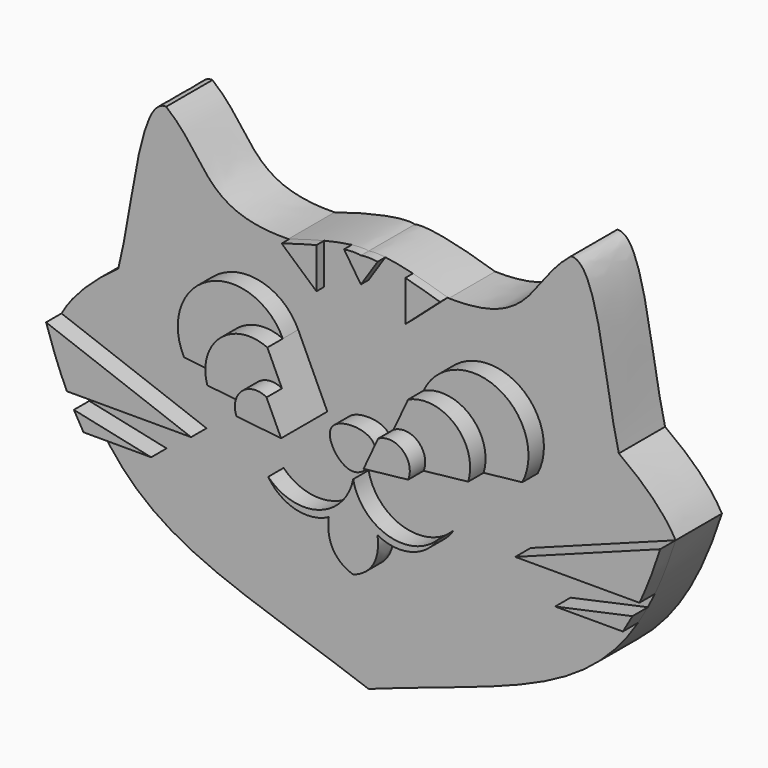
from build123d import *

# Parameters (mm, degrees)
F1_DEPTH       = 7.62
F3_DEPTH       = 2.54
F5_DEPTH       = 2.54
F7_DEPTH       = 2.54
F9_DEPTH       = 2.54
F10_DEPTH      = 1.27
F11_R          = 6.1705322235
F12_DEPTH      = 25.4
F12_DEPTH_BACK = 40.9956
F15_DEPTH      = 2.54
F16_DEPTH      = 2.54
F17_DEPTH      = 2.54


# Not quite as in the source:
# - a feature of the source that left no trace in its solid (it failed there, or was rolled back) is left out


with BuildPart() as f1:
    # F0 (on Front) → F1 (new body)
    with BuildSketch(Plane.XZ):
        with BuildLine():
            add(Edge.make_bspline(
                [(0, 20.3936955137), (1.3948995364, 20.766500107), (5.4805992876, 19.9818174569), (10.5812398311, 18.3488156712)],
                knots=[0, 0, 0, 0, 14.7407470762, 14.7407470762, 14.7407470762, 14.7407470762], degree=3))
            add(Edge.make_bspline(
                [(0, 20.3936955137), (-1.3948995364, 20.766500107), (-5.4805992876, 19.9818174569), (-10.5812398311, 18.3488156712)],
                knots=[0, 0, 0, 0, 14.7407470762, 14.7407470762, 14.7407470762, 14.7407470762], degree=3))
            add(Edge.make_bspline(
                [(-10.5812398311, 18.3488156712), (-17.5782727848, 16.1086720636), (-26.4852430335, 12.2721433588), (-32.9759645779, 7.637338707)],
                knots=[14.7407470762, 14.7407470762, 14.7407470762, 14.7407470762, 34.9620295163, 34.9620295163, 34.9620295163, 34.9620295163], degree=3))
            add(Edge.make_bspline(
                [(-32.9759645779, 7.637338707), (-36.2982275011, 5.2650231569), (-38.9874613211, 2.6835685783), (-40.4635321278, 0)],
                knots=[34.9620295163, 34.9620295163, 34.9620295163, 34.9620295163, 45.3122527465, 45.3122527465, 45.3122527465, 45.3122527465], degree=3))
            add(Edge.make_bspline(
                [(-40.4635321278, 0), (-33.4182982388, -22.0806543438), (-22.6069154368, -22.2432924496), (0, -30.4063044863)],
                knots=[0, 0, 0, 0, 50.6146301455, 50.6146301455, 50.6146301455, 50.6146301455], degree=3))
            add(Edge.make_bspline(
                [(40.4635321278, 0), (33.4182982388, -22.0806543438), (22.6069154368, -22.2432924496), (0, -30.4063044863)],
                knots=[0, 0, 0, 0, 50.6146301455, 50.6146301455, 50.6146301455, 50.6146301455], degree=3))
            add(Edge.make_bspline(
                [(32.9759645779, 7.637338707), (36.2982275011, 5.2650231569), (38.9874613211, 2.6835685783), (40.4635321278, 0)],
                knots=[34.9620295163, 34.9620295163, 34.9620295163, 34.9620295163, 45.3122527465, 45.3122527465, 45.3122527465, 45.3122527465], degree=3))
            add(Edge.make_bspline(
                [(10.5812398311, 18.3488156712), (17.5782727848, 16.1086720636), (26.4852430335, 12.2721433588), (32.9759645779, 7.637338707)],
                knots=[14.7407470762, 14.7407470762, 14.7407470762, 14.7407470762, 34.9620295163, 34.9620295163, 34.9620295163, 34.9620295163], degree=3))
        make_face()
        with BuildLine():
            add(Edge.make_bspline(
                [(-10.5812398311, 18.3488156712), (-17.5782727848, 16.1086720636), (-26.4852430335, 12.2721433588), (-32.9759645779, 7.637338707)],
                knots=[14.7407470762, 14.7407470762, 14.7407470762, 14.7407470762, 34.9620295163, 34.9620295163, 34.9620295163, 34.9620295163], degree=3))
            add(Edge.make_bspline(
                [(-26.6729070635, 28.4619446353), (-21.143157325, 24.0706735486), (-21.7953124032, 18.1571517645), (-10.5812398311, 18.3488156712)],
                knots=[0, 0, 0, 0, 19.0057131348, 19.0057131348, 19.0057131348, 19.0057131348], degree=3))
            add(Edge.make_bspline(
                [(-32.9759645779, 7.637338707), (-31.0729775939, 15.0011911106), (-30.2509800414, 28.7872230125), (-26.6729070635, 28.4619446353)],
                knots=[0, 0, 0, 0, 21.7575905399, 21.7575905399, 21.7575905399, 21.7575905399], degree=3))
        make_face()
        with BuildLine():
            add(Edge.make_bspline(
                [(26.6729070635, 28.4619446353), (21.143157325, 24.0706735486), (21.7953124032, 18.1571517645), (10.5812398311, 18.3488156712)],
                knots=[0, 0, 0, 0, 19.0057131348, 19.0057131348, 19.0057131348, 19.0057131348], degree=3))
            add(Edge.make_bspline(
                [(10.5812398311, 18.3488156712), (17.5782727848, 16.1086720636), (26.4852430335, 12.2721433588), (32.9759645779, 7.637338707)],
                knots=[14.7407470762, 14.7407470762, 14.7407470762, 14.7407470762, 34.9620295163, 34.9620295163, 34.9620295163, 34.9620295163], degree=3))
            add(Edge.make_bspline(
                [(32.9759645779, 7.637338707), (31.0729775939, 15.0011911106), (30.2509800414, 28.7872230125), (26.6729070635, 28.4619446353)],
                knots=[0, 0, 0, 0, 21.7575905399, 21.7575905399, 21.7575905399, 21.7575905399], degree=3))
        make_face()
    extrude(amount=F1_DEPTH)

    # F2 (on face) → F3 (join)
    with BuildSketch(Plane.XZ.offset(7.62)):
        with BuildLine():
            Line((-22.2900346122, 1.8519903891), (-5.4355557593, 0))
            Line((-5.4355557593, 0), (-9.2711227015, 8.2497525646))
            ThreePointArc((-9.2711227015, 8.2497525646), (-19.0491804333, 11.7022032129), (-22.2900346122, 1.8519903891))
        make_face()
        with BuildLine():
            Line((9.2711227015, 8.2497525646), (5.4355557593, 0))
            Line((5.4355557593, 0), (22.2900346122, 1.8519903891))
            ThreePointArc((22.2900346122, 1.8519903891), (19.0491804333, 11.7022032129), (9.2711227015, 8.2497525646))
        make_face()
        with BuildLine():
            add(Edge.make_bspline(
                [(-2.8783681854, 0), (-2.0189454867, 1.4877631411), (5.432970272, 1.496369958), (0.0323743257, -6.8934681979), (-3.6948527353, -1.4134320869), (-2.8783681854, 0)],
                knots=[0, 0, 0, 0, 0.3458251097, 0.6714528725, 1, 1, 1, 1], degree=3))
        make_face()
    extrude(amount=F3_DEPTH)

    # F4 (on face) → F5 (join)
    with BuildSketch(Plane.XZ.offset(10.16)):
        with BuildLine():
            Line((-5.4355557593, 0), (-9.2711227015, 8.2497525646))
            ThreePointArc((-9.2711227015, 8.2497525646), (-15.4885144267, 7.3406406044), (-17.1882661896, 1.2914019444))
            Line((-17.1882661896, 1.2914019444), (-5.4355557593, 0))
        make_face()
        with BuildLine():
            ThreePointArc((17.1882661896, 1.2914019444), (15.4885144267, 7.3406406044), (9.2711227015, 8.2497525646))
            Line((9.2711227015, 8.2497525646), (5.4355557593, 0))
            Line((5.4355557593, 0), (17.1882661896, 1.2914019444))
        make_face()
    extrude(amount=F5_DEPTH)

    # F6 (on face) → F7 (join)
    with BuildSketch(Plane.XZ.offset(12.7)):
        with BuildLine():
            Line((-5.4355557593, 0), (-7.3533392304, 4.1248762823))
            ThreePointArc((-7.3533392304, 4.1248762823), (-10.5856202932, 3.810934338), (-11.3119109744, 0.6457009722))
            Line((-11.3119109744, 0.6457009722), (-5.4355557593, 0))
        make_face()
        with BuildLine():
            ThreePointArc((11.3119109744, 0.6457009722), (10.5856202932, 3.810934338), (7.3533392304, 4.1248762823))
            Line((7.3533392304, 4.1248762823), (5.4355557593, 0))
            Line((5.4355557593, 0), (11.3119109744, 0.6457009722))
        make_face()
    extrude(amount=F7_DEPTH)

    # F8 (on face) → F9 (join)
    with BuildSketch(Plane.XZ.offset(7.62)):
        with BuildLine():
            Line((-21.3572401553, -7.1081966162), (-40.4635321278, 0))
            add(Edge.make_bspline(
                [(-40.4635321278, 0), (-39.6107011325, -2.672880236), (-38.7026836681, -5.0245894415), (-37.7252372782, -7.1081966162)],
                knots=[0, 0, 0, 0, 6.1269400111, 6.1269400111, 6.1269400111, 6.1269400111], degree=3))
            Line((-37.7252372782, -7.1081966162), (-21.3572401553, -7.1081966162))
        make_face()
        with BuildLine():
            Line((-26.6165062785, -11.1537864432), (-36.8009471444, -8.960497845))
            add(Edge.make_bspline(
                [(-36.8009471444, -8.960497845), (-36.3917657951, -9.730841744), (-35.9707421959, -10.4608013384), (-35.5369612337, -11.1537864432)],
                knots=[8.0159459572, 8.0159459572, 8.0159459572, 8.0159459572, 10.4699405675, 10.4699405675, 10.4699405675, 10.4699405675], degree=3))
            Line((-35.5369612337, -11.1537864432), (-26.6165062785, -11.1537864432))
        make_face()
        with BuildLine():
            Line((21.3572401553, -7.1081966162), (37.7252372782, -7.1081966162))
            add(Edge.make_bspline(
                [(40.4635321278, 0), (39.6107011325, -2.672880236), (38.7026836681, -5.0245894415), (37.7252372782, -7.1081966162)],
                knots=[0, 0, 0, 0, 6.1269400111, 6.1269400111, 6.1269400111, 6.1269400111], degree=3))
            Line((40.4635321278, 0), (21.3572401553, -7.1081966162))
        make_face()
        with BuildLine():
            Line((26.6165062785, -11.1537864432), (35.5369612337, -11.1537864432))
            add(Edge.make_bspline(
                [(36.8009471444, -8.960497845), (36.3917657951, -9.730841744), (35.9707421959, -10.4608013384), (35.5369612337, -11.1537864432)],
                knots=[8.0159459572, 8.0159459572, 8.0159459572, 8.0159459572, 10.4699405675, 10.4699405675, 10.4699405675, 10.4699405675], degree=3))
            Line((36.8009471444, -8.960497845), (26.6165062785, -11.1537864432))
        make_face()
    extrude(amount=F9_DEPTH)

    # F8 (on face) → F10 (join)
    with BuildSketch(Plane.XZ.offset(7.62)):
        with BuildLine():
            add(Edge.make_bspline(
                [(-5.8491476811, 19.6953436369), (-7.2292698962, 19.3598221932), (-8.7773553736, 18.9229379667), (-10.4351941553, 18.3954297237)],
                knots=[9.7902198602, 9.7902198602, 9.7902198602, 9.7902198602, 14.5997877749, 14.5997877749, 14.5997877749, 14.5997877749], degree=3))
            Line((-10.4351941553, 18.3954297237), (-5.8491476811, 14.3334269524))
            Line((-5.8491476811, 14.3334269524), (-5.8491476811, 19.6953436369))
        make_face()
        with BuildLine():
            add(Edge.make_bspline(
                [(0, 20.3936955137), (-0.462950485, 20.5174249026), (-1.2222917437, 20.5136574459), (-2.2167587778, 20.3936955137)],
                knots=[0, 0, 0, 0, 4.89227778, 4.89227778, 4.89227778, 4.89227778], degree=3))
            Line((-2.2167587778, 20.3936955137), (0, 17.030486837))
            Line((0, 17.030486837), (2.2167587778, 20.3936955137))
            add(Edge.make_bspline(
                [(2.2167587778, 20.3936955137), (1.2222917437, 20.5136574459), (0.462950485, 20.5174249026), (0, 20.3936955137)],
                knots=[75.3820044828, 75.3820044828, 75.3820044828, 75.3820044828, 80.2742822628, 80.2742822628, 80.2742822628, 80.2742822628], degree=3))
        make_face()
        with BuildLine():
            add(Edge.make_bspline(
                [(10.4351941553, 18.3954297237), (8.7773553736, 18.9229379667), (7.2292698962, 19.3598221932), (5.8491476811, 19.6953436369)],
                knots=[65.674494488, 65.674494488, 65.674494488, 65.674494488, 70.4840624026, 70.4840624026, 70.4840624026, 70.4840624026], degree=3))
            Line((5.8491476811, 19.6953436369), (5.8491476811, 14.3334269524))
            Line((5.8491476811, 14.3334269524), (10.4351941553, 18.3954297237))
        make_face()
    extrude(amount=F10_DEPTH)

    # F11 (on face) → F12 (cut, two sides)
    with BuildSketch(Plane.XZ.offset(7.62)) as f12_sk:
        with Locations((43.2844385505, 30.9309717268)):
            Circle(F11_R)
    extrude(amount=-F12_DEPTH, mode=Mode.SUBTRACT)
    extrude(f12_sk.sketch, amount=F12_DEPTH_BACK, mode=Mode.SUBTRACT)

    # F13 (on face) → F15 (join)
    with BuildSketch(Plane.XZ.offset(7.62)):
        with BuildLine():
            ThreePointArc((0, -5.1889703591), (-0.8834091513, -8.2735351808), (-3.2134445953, -10.4794106752))
            add(Edge.make_bspline(
                [(-3.2134445953, -10.4794106752), (-3.6619147286, -13.9439078048), (-1.7835922772, -15.5332572758), (0, -16.0904042423)],
                knots=[0, 0, 0, 0, 6.4660246656, 6.4660246656, 6.4660246656, 6.4660246656], degree=3))
            add(Edge.make_bspline(
                [(3.2134445953, -10.4794106752), (3.6619147286, -13.9439078048), (1.7835922772, -15.5332572758), (0, -16.0904042423)],
                knots=[0, 0, 0, 0, 6.4660246656, 6.4660246656, 6.4660246656, 6.4660246656], degree=3))
            ThreePointArc((3.2134445953, -10.4794106752), (0.8834091513, -8.2735351808), (0, -5.1889703591))
        make_face()
        with BuildLine():
            ThreePointArc((0, -5.1889703591), (0.0004389266, -5.1159000653), (0, -5.0428297715))
            ThreePointArc((0, -5.0428297715), (-0.0004389266, -5.1159000653), (0, -5.1889703591))
        make_face()
    extrude(amount=F15_DEPTH)

    # F13 (on face) → F16 (join)
    with BuildSketch(Plane.XZ.offset(7.62)):
        with BuildLine():
            ThreePointArc((11.1972401553, -8.4067449109), (4.5859583479, -10.0955669578), (0, -5.0428297715))
            ThreePointArc((0, -5.0428297715), (0.0004389266, -5.1159000653), (0, -5.1889703591))
            ThreePointArc((0, -5.1889703591), (0.8834091513, -8.2735351808), (3.2134445953, -10.4794106752))
            ThreePointArc((3.2134445953, -10.4794106752), (7.6103513449, -11.0031502701), (11.1972401553, -8.4067449109))
        make_face()
    extrude(amount=F16_DEPTH)

    # F13 (on face) → F17 (join)
    with BuildSketch(Plane.XZ.offset(7.62)):
        with BuildLine():
            ThreePointArc((0, -5.0428297715), (-4.5859583479, -10.0955669578), (-11.1972401553, -8.4067449109))
            ThreePointArc((-11.1972401553, -8.4067449109), (-7.6103513449, -11.0031502701), (-3.2134445953, -10.4794106752))
            ThreePointArc((-3.2134445953, -10.4794106752), (-0.8834091513, -8.2735351808), (0, -5.1889703591))
            ThreePointArc((0, -5.1889703591), (-0.0004389266, -5.1159000653), (0, -5.0428297715))
        make_face()
    extrude(amount=F17_DEPTH)


solid = f1.part
